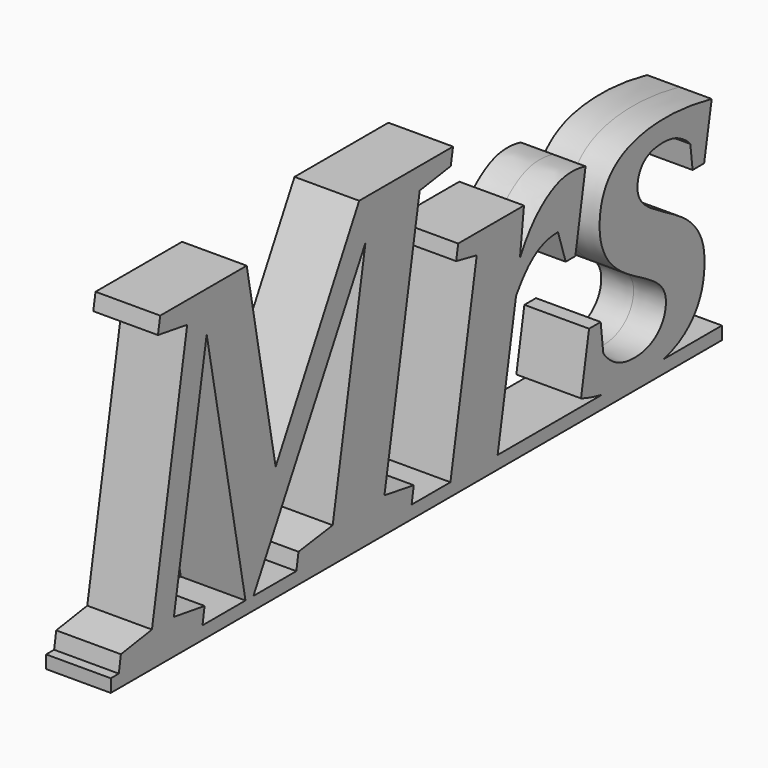
from build123d import *

# Parameters (mm, degrees)
F0_W         = 150
F0_H         = 2.54
F1_DEPTH     = 6.35
F2_TEXT_SIZE = 88.1944444444
F3_DEPTH     = 6.35


# Not quite as in the source:
# - Text() gives the source's letters only with a copy of the font that has no kerning and outlines rounded to 1/6400 em; it was checked with that copy


with BuildPart() as f1:
    # F0 (on Right) → F1 (new body, symmetric)
    with BuildSketch(Plane.YZ):
        with Locations((-5.3918410344, -1.27)):
            Rectangle(F0_W, F0_H)
    extrude(amount=F1_DEPTH, both=True)

    # F2 (on Right) → F3 (join, symmetric)
    with BuildSketch(Plane.YZ):
        with Locations((-77.2574018308, 0)):
            Text('Mrs', F2_TEXT_SIZE, font='Tinos', font_style=FontStyle.BOLDITALIC, text_align=(TextAlign.LEFT, TextAlign.BOTTOM))
    extrude(amount=F3_DEPTH, both=True)


solid = f1.part
